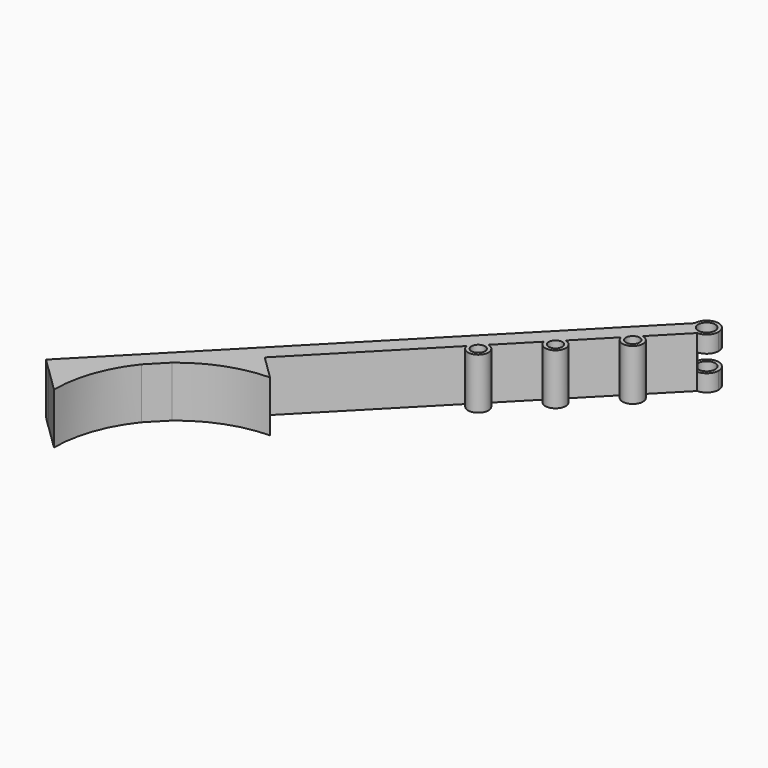
from build123d import *

# Parameters (mm, degrees)
F1_DEPTH  = 15
F2_DEPTH  = 15
F3_W      = 7.4589547733
F3_H      = 5.06
F4_DEPTH  = 25
F5_W      = 8.8782840291
F5_H      = 5.06
F6_DEPTH  = 25
F7_W      = 4.8981418308
F7_H      = 5.06
F8_DEPTH  = 25
F9_DEPTH  = 25
F10_DEPTH = 25
F11_R     = 2.5
F12_DEPTH = 25
F14_DEPTH = 15
F11_R_2   = 2
F15_DEPTH = 25


with BuildPart() as f1:
    # F0 (on Top) → F1 (new body)
    with BuildSketch(Plane.XY):
        with BuildLine():
            ThreePointArc((0, -3.5), (2.4748737342, -2.4748737342), (3.5, 0))
            ThreePointArc((3.5, 0), (0, 3.5), (-3.5, 0))
            ThreePointArc((-3.5, 0), (-2.4748737342, -2.4748737342), (0, -3.5))
        make_face()
    extrude(amount=F1_DEPTH)

    # F0 (on Top) → F2 (join)
    with BuildSketch(Plane.XY):
        with BuildLine():
            ThreePointArc((0, -3.5), (2.4748737342, -2.4748737342), (3.5, 0))
            ThreePointArc((3.5, 0), (0, 3.5), (-3.5, 0))
            ThreePointArc((-3.5, 0), (-2.4748737342, -2.4748737342), (0, -3.5))
        make_face()
        with BuildLine():
            ThreePointArc((0, -3.5), (-2.4748737342, -2.4748737342), (-3.5, 0))
            Line((-3.5, 0), (-108.4601820875, -107.1604412839))
            Line((-108.4601820875, -107.1604412839), (-104.9242736666, -110.6956006351))
            Line((-104.9242736666, -110.6956006351), (-37.3017297765, -41.6092114188))
            Line((-37.3017297765, -41.6092114188), (-33.8042539876, -38.0360247309))
            Line((-33.8042539876, -38.0360247309), (-24.8042539876, -28.8411990533))
            Line((-24.8042539876, -28.8411990533), (-21.3067781987, -25.2680123655))
            Line((-21.3067781987, -25.2680123655), (-12.3067781987, -16.0731866878))
            Line((-12.3067781987, -16.0731866878), (-8.8093024098, -12.5))
            Line((-8.8093024098, -12.5), (0, -3.5))
        make_face()
        with BuildLine():
            ThreePointArc((-12.3067781987, -16.0731866878), (-7.2290363366, -17.5450603078), (-8.8093024098, -12.5))
            Line((-8.8093024098, -12.5), (-12.3067781987, -16.0731866878))
        make_face()
        with BuildLine():
            Line((-33.8042539876, -38.0360247309), (-37.3017297765, -41.6092114188))
            ThreePointArc((-37.3017297765, -41.6092114188), (-32.2239879144, -43.0810850387), (-33.8042539876, -38.0360247309))
        make_face()
        with BuildLine():
            ThreePointArc((-24.8042539876, -28.8411990533), (-19.7265121255, -30.3130726732), (-21.3067781987, -25.2680123655))
            Line((-21.3067781987, -25.2680123655), (-24.8042539876, -28.8411990533))
        make_face()
    extrude(amount=F2_DEPTH)

    # F3 (on face) → F4 (join)
    with BuildSketch(Plane(origin=(-1.7863004718, 1.7496234668, 0), x_dir=(-0.6997345473, -0.7144029419, 0), z_dir=(-0.7144029419, 0.6997345473, 0))):
        with Locations((6.178548302, 7.5)):
            Rectangle(F3_W, F3_H)
    extrude(amount=F4_DEPTH)

    # F5 (on face) → F6 (cut)
    with BuildSketch(Plane(origin=(-1.7136995282, -1.7496234668, 0), x_dir=(-0.7144029419, 0.6997345473, 0), z_dir=(0.6997345473, 0.7144029419, 0))):
        with Locations((6.9395523112, 7.5)):
            Rectangle(F5_W, F5_H)
    extrude(amount=F6_DEPTH, mode=Mode.SUBTRACT)

    # F7 (on face) → F8 (cut)
    with BuildSketch(Plane(origin=(-1.7863004718, 1.7496234668, 0), x_dir=(-0.6997345473, -0.7144029419, 0), z_dir=(-0.7144029419, 0.6997345473, 0))):
        with Locations((0, 7.5)):
            Rectangle(F7_W, F7_H)
    extrude(amount=-F8_DEPTH, mode=Mode.SUBTRACT)

    # F9 (cut): a face of the model
    f9_faces = [f1.faces().sort_by_distance(p)[0] for p in [
        (1.7136995282, 1.7496234668, 7.5),
    ]]
    extrude(f9_faces, amount=-F9_DEPTH, mode=Mode.SUBTRACT)

    # F10 (cut): a face of the model
    f10_faces = [f1.faces().sort_by_distance(p)[0] for p in [
        (-23.9697177179, 14.8290140645, 7.5),
    ]]
    extrude(f10_faces, amount=-F10_DEPTH, mode=Mode.SUBTRACT)

    # F11 (on face) → F12 (cut)
    with BuildSketch(Plane(origin=(0, 0, 0), x_dir=(1, 0, 0), z_dir=(0, 0, -1))):
        Circle(F11_R)
    extrude(amount=-F12_DEPTH, mode=Mode.SUBTRACT)

    # F13 (on face) → F14 (join)
    with BuildSketch(Plane.XY.offset(15)):
        with BuildLine():
            Line((-89.8873776378, -95.3331964442), (-104.8883679048, -110.6589176106))
            Line((-104.8883679048, -110.6589176106), (-97.7441379591, -117.6564594926))
            ThreePointArc((-97.7441379591, -117.6564594926), (-95.7182525009, -105.8252374674), (-89.8873776378, -95.3331964442))
        make_face()
        with BuildLine():
            Line((-62.7933306081, -81.9729853935), (-69.9495157778, -74.9637337568))
            Line((-69.9495157778, -74.9637337568), (-84.9671665368, -90.3064760697))
            ThreePointArc((-84.9671665368, -90.3064760697), (-74.5911866059, -84.2480596514), (-62.7933306081, -81.9729853935))
        make_face()
    extrude(amount=-F14_DEPTH)

    # F11 (on face) → F15 (cut)
    with BuildSketch(Plane(origin=(0, 0, 0), x_dir=(1, 0, 0), z_dir=(0, 0, -1))):
        Circle(F11_R)
        with Locations((-34.3678999271, 40.9825995654)):
            Circle(F11_R_2)
        with Locations((-21.8704241382, 28.2145871999)):
            Circle(F11_R_2)
        with Locations((-9.3729483493, 15.4465748344)):
            Circle(F11_R_2)
    extrude(amount=-F15_DEPTH, mode=Mode.SUBTRACT)


solid = f1.part
